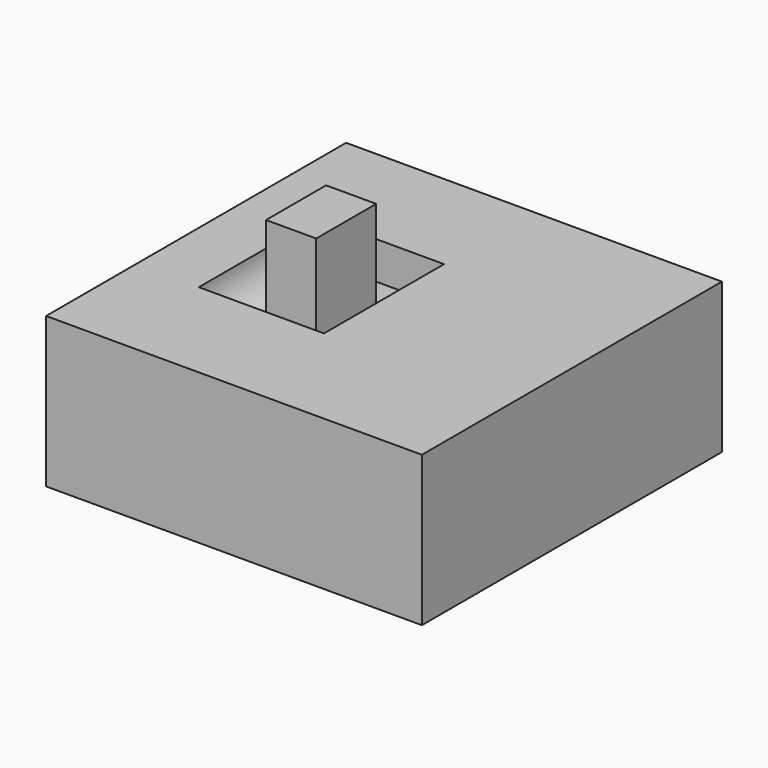
from build123d import *

# Parameters (mm, degrees)
F0_W          = 127.2562742233
F0_H          = 50.8075356483
F1_DEPTH      = 63.5
F1_DEPTH_BACK = 63.5
F3_DEPTH      = 12.7
F4_R          = 12.69999
F5_W          = 16.97918742
F5_H          = 25.4037678242
F6_DEPTH      = 31.75


# Not quite as in the source:
# - a fillet or chamfer is up to 0.001 mm smaller than in the source, because OpenCascade refuses the exact size


with BuildPart() as f1:
    # F0 (on Front) → F1 (new body, two sides)
    with BuildSketch(Plane.XZ) as f1_sk:
        with Locations((0, 25.4037678242)):
            Rectangle(F0_W, F0_H)
    extrude(amount=F1_DEPTH)
    extrude(f1_sk.sketch, amount=-F1_DEPTH_BACK)

    # F2 (on face) → F3 (cut)
    with BuildSketch(Plane.XY.offset(50.8075356483)):
        Polygon((0, -25.4037678242), (0, 0), (0, 25.4037678242), (-42.37918742, 25.4037678242), (-42.37918742, 0), (-42.37918742, -25.4037678242), align=None)
    extrude(amount=-F3_DEPTH, mode=Mode.SUBTRACT)

    # F4 (radius 12.7 in the source; OpenCascade refuses exactly that, so slightly less here)
    f4_edges = [f1.edges().sort_by_distance(p)[0] for p in [
        (-42.379187, 0, 38.107536),
        (0, 0, 38.107536),
    ]]
    fillet(f4_edges, radius=F4_R)

    # F5 (on face) → F6 (join)
    with BuildSketch(Plane.XY.offset(38.1075356483)):
        with Locations((-21.18959371, -0.1187091693)):
            Rectangle(F5_W, F5_H)
    extrude(amount=F6_DEPTH)


solid = f1.part
